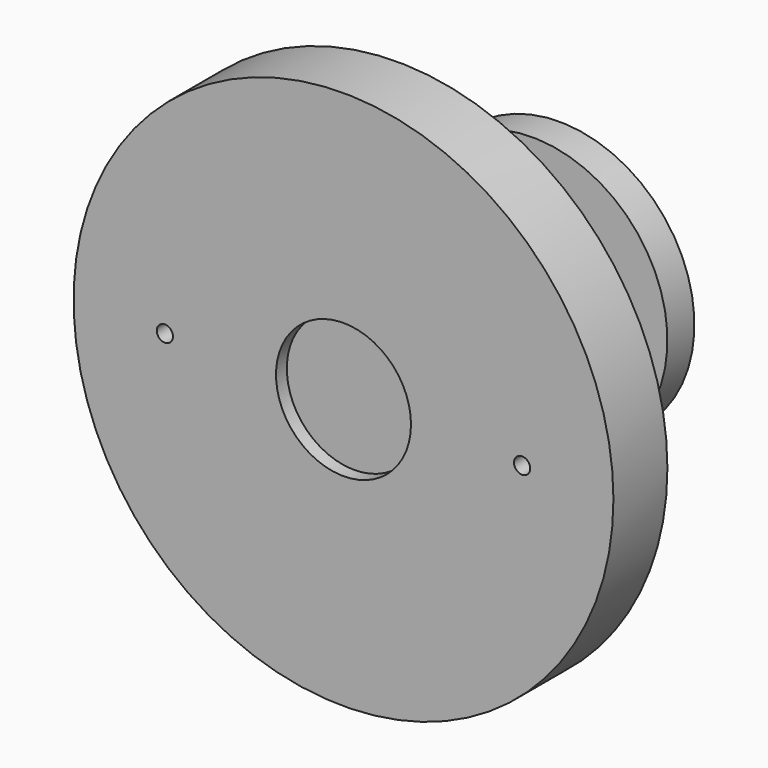
from build123d import *

# Parameters (mm, degrees)
F0_R          = 20
F1_DEPTH      = 5
F2_R          = 0.6
F3_DEPTH      = 5
F4_R          = 2.5
F5_DEPTH      = 15
F6_R          = 1
F7_DEPTH      = 25
F7_DEPTH_BACK = 25
F9_DEPTH      = 25
F9_DEPTH_BACK = 25
F8_R          = 5
F10_DEPTH     = 1
F11_R         = 10
F12_DEPTH     = 2.5


# Not quite as in the source:
# - a feature names something its author has since deleted; it is built from what else it names


with BuildPart() as f1:
    # F0 (on Front) → F1 (new body)
    with BuildSketch(Plane.XZ):
        Circle(F0_R)
    extrude(amount=F1_DEPTH)

    # F2 (on face) → F3 (cut, through all)
    with BuildSketch(Plane.XZ.offset(5)):
        with Locations((-13.23387, 0)):
            Circle(F2_R)
        with Locations((13.23387, 0)):
            Circle(F2_R)
    extrude(amount=-F3_DEPTH, mode=Mode.SUBTRACT)

    # F4 (on face) → F5 (join)
    with BuildSketch(Plane.XZ):
        Circle(F4_R)
    extrude(amount=-F5_DEPTH)

    # F6 (on Top) → F7 (cut, two sides)
    with BuildSketch(Plane.XY) as f7_sk:
        with Locations((0, 6.5963385438)):
            Circle(F6_R)
    extrude(amount=F7_DEPTH, mode=Mode.SUBTRACT)
    extrude(f7_sk.sketch, amount=-F7_DEPTH_BACK, mode=Mode.SUBTRACT)

    # F6 (on Top) → F9 (cut, two sides)
    with BuildSketch(Plane.XY) as f9_sk:
        with Locations((0, 6.5963385438)):
            Circle(F6_R)
    extrude(amount=-F9_DEPTH, mode=Mode.SUBTRACT)
    extrude(f9_sk.sketch, amount=F9_DEPTH_BACK, mode=Mode.SUBTRACT)

    # F8 (on face) → F10 (cut)
    with BuildSketch(Plane.XZ.offset(5)):
        Circle(F8_R)
    extrude(amount=-F10_DEPTH, mode=Mode.SUBTRACT)

    # F11 (on face) → F12 (join)
    with BuildSketch(Plane(origin=(0, 15, 0), x_dir=(-1, 0, 0), z_dir=(0, 1, 0))):
        Circle(F11_R)
    extrude(amount=-F12_DEPTH)


solid = f1.part
